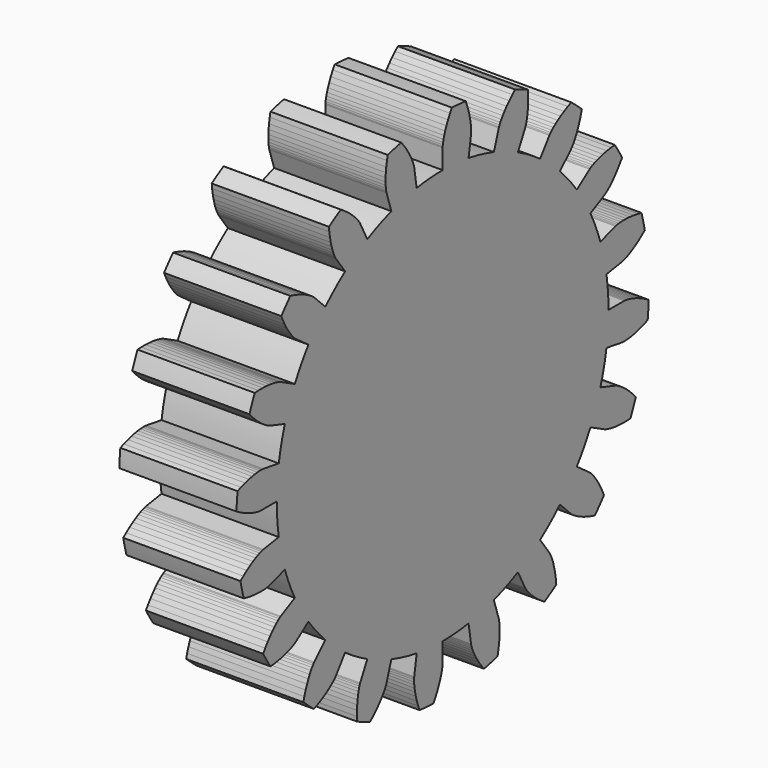
from build123d import *

# Parameters (mm, degrees)
F2_DEPTH = 12.7


# Not quite as in the source:
# - a variable given as a bare number and used for a length is read in inches; the dataset says mm whatever the document's units were


with BuildPart() as f2:
    # F1 (on Right) → F2 (new body)
    with BuildSketch(Plane.YZ):
        with BuildLine():
            ThreePointArc((22.1846851095, -3.5137089349), (22.3919795548, -1.7622870101), (22.46122, 0))
            ThreePointArc((22.46122, 0), (22.3919795548, 1.7622870101), (22.1846851095, 3.5137089349))
            ThreePointArc((22.1846851095, 3.5137089349), (21.8406147034, 5.2434676755), (21.3618896449, 6.9408986944))
            ThreePointArc((21.3618896449, 6.9408986944), (20.7514614332, 8.5955367647), (20.0130935612, 10.1971804926))
            ThreePointArc((20.0130935612, 10.1971804926), (19.1513383124, 11.7359552118), (18.1715086944, 13.2023738645))
            ThreePointArc((18.1715086944, 13.2023738645), (17.0796456827, 14.5873954921), (15.8824809757, 15.8824809757))
            ThreePointArc((15.8824809757, 15.8824809757), (14.5873954921, 17.0796456827), (13.2023738645, 18.1715086944))
            ThreePointArc((13.2023738645, 18.1715086944), (11.7359552118, 19.1513383124), (10.1971804926, 20.0130935612))
            ThreePointArc((10.1971804926, 20.0130935612), (8.5955367647, 20.7514614332), (6.9408986944, 21.3618896449))
            ThreePointArc((6.9408986944, 21.3618896449), (5.2434676755, 21.8406147034), (3.5137089349, 22.1846851095))
            ThreePointArc((3.5137089349, 22.1846851095), (1.7622870101, 22.3919795548), (0, 22.46122))
            ThreePointArc((0, 22.46122), (-1.7622870101, 22.3919795548), (-3.5137089349, 22.1846851095))
            ThreePointArc((-3.5137089349, 22.1846851095), (-5.2434676755, 21.8406147034), (-6.9408986944, 21.3618896449))
            ThreePointArc((-6.9408986944, 21.3618896449), (-8.5955367647, 20.7514614332), (-10.1971804926, 20.0130935612))
            ThreePointArc((-10.1971804926, 20.0130935612), (-11.7359552118, 19.1513383124), (-13.2023738645, 18.1715086944))
            ThreePointArc((-13.2023738645, 18.1715086944), (-14.5873954921, 17.0796456827), (-15.8824809757, 15.8824809757))
            ThreePointArc((-15.8824809757, 15.8824809757), (-17.0796456827, 14.5873954921), (-18.1715086944, 13.2023738645))
            ThreePointArc((-18.1715086944, 13.2023738645), (-19.1513383124, 11.7359552118), (-20.0130935612, 10.1971804926))
            ThreePointArc((-20.0130935612, 10.1971804926), (-20.7514614332, 8.5955367647), (-21.3618896449, 6.9408986944))
            ThreePointArc((-21.3618896449, 6.9408986944), (-21.8406147034, 5.2434676755), (-22.1846851095, 3.5137089349))
            ThreePointArc((-22.1846851095, 3.5137089349), (-22.3919795548, 1.7622870101), (-22.46122, 0))
            ThreePointArc((-22.46122, 0), (-22.3919795548, -1.7622870101), (-22.1846851095, -3.5137089349))
            ThreePointArc((-22.1846851095, -3.5137089349), (-21.8406147034, -5.2434676755), (-21.3618896449, -6.9408986944))
            ThreePointArc((-21.3618896449, -6.9408986944), (-20.7514614332, -8.5955367647), (-20.0130935612, -10.1971804926))
            ThreePointArc((-20.0130935612, -10.1971804926), (-19.1513383124, -11.7359552118), (-18.1715086944, -13.2023738645))
            ThreePointArc((-18.1715086944, -13.2023738645), (-17.0796456827, -14.5873954921), (-15.8824809757, -15.8824809757))
            ThreePointArc((-15.8824809757, -15.8824809757), (-14.5873954921, -17.0796456827), (-13.2023738645, -18.1715086944))
            ThreePointArc((-13.2023738645, -18.1715086944), (-11.7359552118, -19.1513383124), (-10.1971804926, -20.0130935612))
            ThreePointArc((-10.1971804926, -20.0130935612), (-8.5955367647, -20.7514614332), (-6.9408986944, -21.3618896449))
            ThreePointArc((-6.9408986944, -21.3618896449), (-5.2434676755, -21.8406147034), (-3.5137089349, -22.1846851095))
            ThreePointArc((-3.5137089349, -22.1846851095), (-1.7622870101, -22.3919795548), (0, -22.46122))
            ThreePointArc((0, -22.46122), (1.7622870101, -22.3919795548), (3.5137089349, -22.1846851095))
            ThreePointArc((3.5137089349, -22.1846851095), (5.2434676755, -21.8406147034), (6.9408986944, -21.3618896449))
            ThreePointArc((6.9408986944, -21.3618896449), (8.5955367647, -20.7514614332), (10.1971804926, -20.0130935612))
            ThreePointArc((10.1971804926, -20.0130935612), (11.7359552118, -19.1513383124), (13.2023738645, -18.1715086944))
            ThreePointArc((13.2023738645, -18.1715086944), (14.5873954921, -17.0796456827), (15.8824809757, -15.8824809757))
            ThreePointArc((15.8824809757, -15.8824809757), (17.0796456827, -14.5873954921), (18.1715086944, -13.2023738645))
            ThreePointArc((18.1715086944, -13.2023738645), (19.1513383124, -11.7359552118), (20.0130935612, -10.1971804926))
            ThreePointArc((20.0130935612, -10.1971804926), (20.7514614332, -8.5955367647), (21.3618896449, -6.9408986944))
            ThreePointArc((21.3618896449, -6.9408986944), (21.8406147034, -5.2434676755), (22.1846851095, -3.5137089349))
        make_face()
        with BuildLine():
            Line((-23.3873833018, -7.5990214781), (-21.3618896449, -6.9408986944))
            ThreePointArc((-21.3618896449, -6.9408986944), (-21.8406147034, -5.2434676755), (-22.1846851095, -3.5137089349))
            Line((-22.1846851095, -3.5137089349), (-24.288194664, -3.8468721183))
            Line((-24.288194664, -3.8468721183), (-24.3183756913, -3.8526894407))
            Line((-24.3183756913, -3.8526894407), (-24.4080512003, -3.8741463554))
            Line((-24.4080512003, -3.8741463554), (-24.5555837939, -3.9171690334))
            Line((-24.5555837939, -3.9171690334), (-24.7588943631, -3.987551636))
            Line((-24.7588943631, -3.987551636), (-25.0154715589, -4.0909270813))
            Line((-25.0154715589, -4.0909270813), (-25.3223830759, -4.2327384457))
            Line((-25.3223830759, -4.2327384457), (-25.6762887078, -4.4182111085))
            Line((-25.6762887078, -4.4182111085), (-26.0734551281, -4.6523257442))
            Line((-26.0734551281, -4.6523257442), (-26.5097723413, -4.939792266))
            Line((-26.5097723413, -4.939792266), (-26.9807717473, -5.2850248183))
            Line((-26.9807717473, -5.2850248183), (-27.3723694253, -5.6033018877))
            ThreePointArc((-27.3723694253, -5.6033018877), (-27.1680155759, -6.5224634661), (-26.9328055646, -7.4342171355))
            Line((-26.9328055646, -7.4342171355), (-26.4393947129, -7.5400224553))
            Line((-26.4393947129, -7.5400224553), (-25.8629988703, -7.633797656))
            Line((-25.8629988703, -7.633797656), (-25.3437303169, -7.6918483328))
            Line((-25.3437303169, -7.6918483328), (-24.8835666247, -7.720136219))
            Line((-24.8835666247, -7.720136219), (-24.4840315708, -7.7247237769))
            Line((-24.4840315708, -7.7247237769), (-24.1461903947, -7.7117437148))
            Line((-24.1461903947, -7.7117437148), (-23.8706469692, -7.6873683017))
            Line((-23.8706469692, -7.6873683017), (-23.6575428926, -7.6577785929))
            Line((-23.6575428926, -7.6577785929), (-23.5065585022, -7.6291336838))
            Line((-23.5065585022, -7.6291336838), (-23.4169158032, -7.6075401056))
            Line((-23.4169158032, -7.6075401056), (-23.3873833018, -7.5990214781))
        make_face()
        with BuildLine():
            Line((-19.8944965109, -14.4541977884), (-18.1715086944, -13.2023738645))
            ThreePointArc((-18.1715086944, -13.2023738645), (-19.1513383124, -11.7359552118), (-20.0130935612, -10.1971804926))
            Line((-20.0130935612, -10.1971804926), (-21.9106969444, -11.1640577094))
            Line((-21.9106969444, -11.1640577094), (-21.9376031557, -11.1789167621))
            Line((-21.9376031557, -11.1789167621), (-22.0162590816, -11.2270347569))
            Line((-22.0162590816, -11.2270347569), (-22.1432761774, -11.3135418337))
            Line((-22.1432761774, -11.3135418337), (-22.3148865988, -11.4433060876))
            Line((-22.3148865988, -11.4433060876), (-22.5269612434, -11.6209086924))
            Line((-22.5269612434, -11.6209086924), (-22.7750293199, -11.8506201891))
            Line((-22.7750293199, -11.8506201891), (-23.0542993726, -12.1363780283))
            Line((-23.0542993726, -12.1363780283), (-23.3596816836, -12.4817654516))
            Line((-23.3596816836, -12.4817654516), (-23.6858119718, -12.8899917942))
            Line((-23.6858119718, -12.8899917942), (-24.0270763004, -13.3638742835))
            Line((-24.0270763004, -13.3638742835), (-24.3011548004, -13.7875841018))
            ThreePointArc((-24.3011548004, -13.7875841018), (-23.8227661921, -14.5986098982), (-23.3173207996, -15.3930552759))
            Line((-23.3173207996, -15.3930552759), (-22.8153635519, -15.3412097764))
            Line((-22.8153635519, -15.3412097764), (-22.2382003992, -15.2522791813))
            Line((-22.2382003992, -15.2522791813), (-21.7264080121, -15.147025848))
            Line((-21.7264080121, -15.147025848), (-21.2800248965, -15.0317308255))
            Line((-21.2800248965, -15.0317308255), (-20.8986268467, -14.9126307308))
            Line((-20.8986268467, -14.9126307308), (-20.5813318544, -14.7958872934))
            Line((-20.5813318544, -14.7958872934), (-20.326806901, -14.6875572967))
            Line((-20.326806901, -14.6875572967), (-20.1332766032, -14.5935630301))
            Line((-20.1332766032, -14.5935630301), (-19.9985336785, -14.5196633601))
            Line((-19.9985336785, -14.5196633601), (-19.9199511881, -14.4714255295))
            Line((-19.9199511881, -14.4714255295), (-19.8944965109, -14.4541977884))
        make_face()
        with BuildLine():
            Line((-14.4541977884, -19.8944965109), (-13.2023738645, -18.1715086944))
            ThreePointArc((-13.2023738645, -18.1715086944), (-14.5873954921, -17.0796456827), (-15.8824809757, -15.8824809757))
            Line((-15.8824809757, -15.8824809757), (-17.3884275472, -17.3884275472))
            Line((-17.3884275472, -17.3884275472), (-17.409425175, -17.4108738227))
            Line((-17.409425175, -17.4108738227), (-17.4693621277, -17.480942773))
            Line((-17.4693621277, -17.480942773), (-17.5634304075, -17.6024663333))
            Line((-17.5634304075, -17.6024663333), (-17.6865422573, -17.7789100092))
            Line((-17.6865422573, -17.7789100092), (-17.8333550069, -18.013354793))
            Line((-17.8333550069, -18.013354793), (-17.9982970112, -18.3084806602))
            Line((-17.9982970112, -18.3084806602), (-18.175594586, -18.6665517076))
            Line((-18.175594586, -18.6665517076), (-18.3592998394, -19.0894029911))
            Line((-18.3592998394, -19.0894029911), (-18.5433192977, -19.5784291157))
            Line((-18.5433192977, -19.5784291157), (-18.7214432188, -20.1345746222))
            Line((-18.7214432188, -20.1345746222), (-18.8511738276, -20.6222415203))
            ThreePointArc((-18.8511738276, -20.6222415203), (-18.1455784703, -21.2457426789), (-17.4193742134, -21.8451139162))
            Line((-17.4193742134, -21.8451139162), (-16.9580056425, -21.6406925961))
            Line((-16.9580056425, -21.6406925961), (-16.4365719304, -21.3777613514))
            Line((-16.4365719304, -21.3777613514), (-15.9823535143, -21.1195069377))
            Line((-15.9823535143, -21.1195069377), (-15.5934460648, -20.8719148865))
            Line((-15.5934460648, -20.8719148865), (-15.2675189175, -20.6407854863))
            Line((-15.2675189175, -20.6407854863), (-15.0018291537, -20.4317063346))
            Line((-15.0018291537, -20.4317063346), (-14.7932373481, -20.2500258493))
            Line((-14.7932373481, -20.2500258493), (-14.6382249231, -20.1008278386))
            Line((-14.6382249231, -20.1008278386), (-14.5329130404, -19.9889072223))
            Line((-14.5329130404, -19.9889072223), (-14.4730829603, -19.9187469941))
            Line((-14.4730829603, -19.9187469941), (-14.4541977884, -19.8944965109))
        make_face()
        with BuildLine():
            Line((-7.5990214781, -23.3873833018), (-6.9408986944, -21.3618896449))
            ThreePointArc((-6.9408986944, -21.3618896449), (-8.5955367647, -20.7514614332), (-10.1971804926, -20.0130935612))
            Line((-10.1971804926, -20.0130935612), (-11.1640577094, -21.9106969444))
            Line((-11.1640577094, -21.9106969444), (-11.1770913595, -21.9385332448))
            Line((-11.1770913595, -21.9385332448), (-11.2124422925, -22.0236943136))
            Line((-11.2124422925, -22.0236943136), (-11.2643536976, -22.1683387846))
            Line((-11.2643536976, -22.1683387846), (-11.3269159302, -22.3741903461))
            Line((-11.3269159302, -22.3741903461), (-11.3940957299, -22.6425282201))
            Line((-11.3940957299, -22.6425282201), (-11.4597659895, -22.9741794817))
            Line((-11.4597659895, -22.9741794817), (-11.5177359646, -23.3695132482))
            Line((-11.5177359646, -23.3695132482), (-11.5617818102, -23.8284367621))
            Line((-11.5617818102, -23.8284367621), (-11.5856773319, -24.3503933845))
            Line((-11.5856773319, -24.3503933845), (-11.5832248349, -24.9343625111))
            Line((-11.5832248349, -24.9343625111), (-11.5559086167, -25.4382502551))
            ThreePointArc((-11.5559086167, -25.4382502551), (-10.6921751003, -25.8131941384), (-9.8162979113, -26.1588206026))
            Line((-9.8162979113, -26.1588206026), (-9.4406799874, -25.8218336449))
            Line((-9.4406799874, -25.8218336449), (-9.0260172807, -25.4106392928))
            Line((-9.0260172807, -25.4106392928), (-8.6738348989, -25.0246635401))
            Line((-8.6738348989, -25.0246635401), (-8.3804720864, -24.6690104953))
            Line((-8.3804720864, -24.6690104953), (-8.1419198617, -24.3484763457))
            Line((-8.1419198617, -24.3484763457), (-7.9538428915, -24.0675276037))
            Line((-7.9538428915, -24.0675276037), (-7.8116026531, -23.8302807815))
            Line((-7.8116026531, -23.8302807815), (-7.710281797, -23.6404835675))
            Line((-7.710281797, -23.6404835675), (-7.6447096172, -23.5014975746))
            Line((-7.6447096172, -23.5014975746), (-7.6094885324, -23.4162827209))
            Line((-7.6094885324, -23.4162827209), (-7.5990214781, -23.3873833018))
        make_face()
        with BuildLine():
            Line((0, -24.5909500656), (0, -22.46122))
            ThreePointArc((0, -22.46122), (-1.7622870101, -22.3919795548), (-3.5137089349, -22.1846851095))
            Line((-3.5137089349, -22.1846851095), (-3.8468721183, -24.288194664))
            Line((-3.8468721183, -24.288194664), (-3.8506659664, -24.3186961782))
            Line((-3.8506659664, -24.3186961782), (-3.8579704841, -24.4106132066))
            Line((-3.8579704841, -24.4106132066), (-3.8626435645, -24.5642197798))
            Line((-3.8626435645, -24.5642197798), (-3.8585321527, -24.7793290418))
            Line((-3.8585321527, -24.7793290418), (-3.8395029756, -25.0552932252))
            Line((-3.8395029756, -25.0552932252), (-3.7994732279, -25.3910055449))
            Line((-3.7994732279, -25.3910055449), (-3.7324410981, -25.7849040071))
            Line((-3.7324410981, -25.7849040071), (-3.6325160217, -26.2349771203))
            Line((-3.6325160217, -26.2349771203), (-3.4939485467, -26.7387714896))
            Line((-3.4939485467, -26.7387714896), (-3.3111596991, -27.2934012695))
            Line((-3.3111596991, -27.2934012695), (-3.1294705556, -27.7641858163))
            ThreePointArc((-3.1294705556, -27.7641858163), (-2.1921471346, -27.8538703045), (-1.2523339754, -27.9119196691))
            Line((-1.2523339754, -27.9119196691), (-0.9992347981, -27.4753537053))
            Line((-0.9992347981, -27.4753537053), (-0.7319331716, -26.9561468139))
            Line((-0.7319331716, -26.9561468139), (-0.5162608895, -26.4802317181))
            Line((-0.5162608895, -26.4802317181), (-0.3471591099, -26.0513314777))
            Line((-0.3471591099, -26.0513314777), (-0.2193329616, -25.6727686945))
            Line((-0.2193329616, -25.6727686945), (-0.1272790694, -25.3474515827))
            Line((-0.1272790694, -25.3474515827), (-0.0653138637, -25.0778617955))
            Line((-0.0653138637, -25.0778617955), (-0.0276025679, -24.8660440519))
            Line((-0.0276025679, -24.8660440519), (-0.0081887528, -24.7135975998))
            Line((-0.0081887528, -24.7135975998), (-0.0010243486, -24.6216695442))
            Line((-0.0010243486, -24.6216695442), (0, -24.5909500656))
        make_face()
        with BuildLine():
            Line((7.5990214781, -23.3873833018), (6.9408986944, -21.3618896449))
            ThreePointArc((6.9408986944, -21.3618896449), (5.2434676755, -21.8406147034), (3.5137089349, -22.1846851095))
            Line((3.5137089349, -22.1846851095), (3.8468721183, -24.288194664))
            Line((3.8468721183, -24.288194664), (3.8526894407, -24.3183756913))
            Line((3.8526894407, -24.3183756913), (3.8741463554, -24.4080512003))
            Line((3.8741463554, -24.4080512003), (3.9171690334, -24.5555837939))
            Line((3.9171690334, -24.5555837939), (3.987551636, -24.7588943631))
            Line((3.987551636, -24.7588943631), (4.0909270813, -25.0154715589))
            Line((4.0909270813, -25.0154715589), (4.2327384457, -25.3223830759))
            Line((4.2327384457, -25.3223830759), (4.4182111085, -25.6762887078))
            Line((4.4182111085, -25.6762887078), (4.6523257442, -26.0734551281))
            Line((4.6523257442, -26.0734551281), (4.939792266, -26.5097723413))
            Line((4.939792266, -26.5097723413), (5.2850248183, -26.9807717473))
            Line((5.2850248183, -26.9807717473), (5.6033018877, -27.3723694253))
            ThreePointArc((5.6033018877, -27.3723694253), (6.5224634661, -27.1680155759), (7.4342171355, -26.9328055646))
            Line((7.4342171355, -26.9328055646), (7.5400224553, -26.4393947129))
            Line((7.5400224553, -26.4393947129), (7.633797656, -25.8629988703))
            Line((7.633797656, -25.8629988703), (7.6918483328, -25.3437303169))
            Line((7.6918483328, -25.3437303169), (7.720136219, -24.8835666247))
            Line((7.720136219, -24.8835666247), (7.7247237769, -24.4840315708))
            Line((7.7247237769, -24.4840315708), (7.7117437148, -24.1461903947))
            Line((7.7117437148, -24.1461903947), (7.6873683017, -23.8706469692))
            Line((7.6873683017, -23.8706469692), (7.6577785929, -23.6575428926))
            Line((7.6577785929, -23.6575428926), (7.6291336838, -23.5065585022))
            Line((7.6291336838, -23.5065585022), (7.6075401056, -23.4169158032))
            Line((7.6075401056, -23.4169158032), (7.5990214781, -23.3873833018))
        make_face()
        with BuildLine():
            Line((14.4541977884, -19.8944965109), (13.2023738645, -18.1715086944))
            ThreePointArc((13.2023738645, -18.1715086944), (11.7359552118, -19.1513383124), (10.1971804926, -20.0130935612))
            Line((10.1971804926, -20.0130935612), (11.1640577094, -21.9106969444))
            Line((11.1640577094, -21.9106969444), (11.1789167621, -21.9376031557))
            Line((11.1789167621, -21.9376031557), (11.2270347569, -22.0162590816))
            Line((11.2270347569, -22.0162590816), (11.3135418337, -22.1432761774))
            Line((11.3135418337, -22.1432761774), (11.4433060876, -22.3148865988))
            Line((11.4433060876, -22.3148865988), (11.6209086924, -22.5269612434))
            Line((11.6209086924, -22.5269612434), (11.8506201891, -22.7750293199))
            Line((11.8506201891, -22.7750293199), (12.1363780283, -23.0542993726))
            Line((12.1363780283, -23.0542993726), (12.4817654516, -23.3596816836))
            Line((12.4817654516, -23.3596816836), (12.8899917942, -23.6858119718))
            Line((12.8899917942, -23.6858119718), (13.3638742835, -24.0270763004))
            Line((13.3638742835, -24.0270763004), (13.7875841018, -24.3011548004))
            ThreePointArc((13.7875841018, -24.3011548004), (14.5986098982, -23.8227661921), (15.3930552759, -23.3173207996))
            Line((15.3930552759, -23.3173207996), (15.3412097764, -22.8153635519))
            Line((15.3412097764, -22.8153635519), (15.2522791813, -22.2382003992))
            Line((15.2522791813, -22.2382003992), (15.147025848, -21.7264080121))
            Line((15.147025848, -21.7264080121), (15.0317308255, -21.2800248965))
            Line((15.0317308255, -21.2800248965), (14.9126307308, -20.8986268467))
            Line((14.9126307308, -20.8986268467), (14.7958872934, -20.5813318544))
            Line((14.7958872934, -20.5813318544), (14.6875572967, -20.326806901))
            Line((14.6875572967, -20.326806901), (14.5935630301, -20.1332766032))
            Line((14.5935630301, -20.1332766032), (14.5196633601, -19.9985336785))
            Line((14.5196633601, -19.9985336785), (14.4714255295, -19.9199511881))
            Line((14.4714255295, -19.9199511881), (14.4541977884, -19.8944965109))
        make_face()
        with BuildLine():
            Line((19.8944965109, -14.4541977884), (18.1715086944, -13.2023738645))
            ThreePointArc((18.1715086944, -13.2023738645), (17.0796456827, -14.5873954921), (15.8824809757, -15.8824809757))
            Line((15.8824809757, -15.8824809757), (17.3884275472, -17.3884275472))
            Line((17.3884275472, -17.3884275472), (17.4108738227, -17.409425175))
            Line((17.4108738227, -17.409425175), (17.480942773, -17.4693621277))
            Line((17.480942773, -17.4693621277), (17.6024663333, -17.5634304075))
            Line((17.6024663333, -17.5634304075), (17.7789100092, -17.6865422573))
            Line((17.7789100092, -17.6865422573), (18.013354793, -17.8333550069))
            Line((18.013354793, -17.8333550069), (18.3084806602, -17.9982970112))
            Line((18.3084806602, -17.9982970112), (18.6665517076, -18.175594586))
            Line((18.6665517076, -18.175594586), (19.0894029911, -18.3592998394))
            Line((19.0894029911, -18.3592998394), (19.5784291157, -18.5433192977))
            Line((19.5784291157, -18.5433192977), (20.1345746222, -18.7214432188))
            Line((20.1345746222, -18.7214432188), (20.6222415203, -18.8511738276))
            ThreePointArc((20.6222415203, -18.8511738276), (21.2457426789, -18.1455784703), (21.8451139162, -17.4193742134))
            Line((21.8451139162, -17.4193742134), (21.6406925961, -16.9580056425))
            Line((21.6406925961, -16.9580056425), (21.3777613514, -16.4365719304))
            Line((21.3777613514, -16.4365719304), (21.1195069377, -15.9823535143))
            Line((21.1195069377, -15.9823535143), (20.8719148865, -15.5934460648))
            Line((20.8719148865, -15.5934460648), (20.6407854863, -15.2675189175))
            Line((20.6407854863, -15.2675189175), (20.4317063346, -15.0018291537))
            Line((20.4317063346, -15.0018291537), (20.2500258493, -14.7932373481))
            Line((20.2500258493, -14.7932373481), (20.1008278386, -14.6382249231))
            Line((20.1008278386, -14.6382249231), (19.9889072223, -14.5329130404))
            Line((19.9889072223, -14.5329130404), (19.9187469941, -14.4730829603))
            Line((19.9187469941, -14.4730829603), (19.8944965109, -14.4541977884))
        make_face()
        with BuildLine():
            Line((23.3873833018, -7.5990214781), (21.3618896449, -6.9408986944))
            ThreePointArc((21.3618896449, -6.9408986944), (20.7514614332, -8.5955367647), (20.0130935612, -10.1971804926))
            Line((20.0130935612, -10.1971804926), (21.9106969444, -11.1640577094))
            Line((21.9106969444, -11.1640577094), (21.9385332448, -11.1770913595))
            Line((21.9385332448, -11.1770913595), (22.0236943136, -11.2124422925))
            Line((22.0236943136, -11.2124422925), (22.1683387846, -11.2643536976))
            Line((22.1683387846, -11.2643536976), (22.3741903461, -11.3269159302))
            Line((22.3741903461, -11.3269159302), (22.6425282201, -11.3940957299))
            Line((22.6425282201, -11.3940957299), (22.9741794817, -11.4597659895))
            Line((22.9741794817, -11.4597659895), (23.3695132482, -11.5177359646))
            Line((23.3695132482, -11.5177359646), (23.8284367621, -11.5617818102))
            Line((23.8284367621, -11.5617818102), (24.3503933845, -11.5856773319))
            Line((24.3503933845, -11.5856773319), (24.9343625111, -11.5832248349))
            Line((24.9343625111, -11.5832248349), (25.4382502551, -11.5559086167))
            ThreePointArc((25.4382502551, -11.5559086167), (25.8131941384, -10.6921751003), (26.1588206026, -9.8162979113))
            Line((26.1588206026, -9.8162979113), (25.8218336449, -9.4406799874))
            Line((25.8218336449, -9.4406799874), (25.4106392928, -9.0260172807))
            Line((25.4106392928, -9.0260172807), (25.0246635401, -8.6738348989))
            Line((25.0246635401, -8.6738348989), (24.6690104953, -8.3804720864))
            Line((24.6690104953, -8.3804720864), (24.3484763457, -8.1419198617))
            Line((24.3484763457, -8.1419198617), (24.0675276037, -7.9538428915))
            Line((24.0675276037, -7.9538428915), (23.8302807815, -7.8116026531))
            Line((23.8302807815, -7.8116026531), (23.6404835675, -7.710281797))
            Line((23.6404835675, -7.710281797), (23.5014975746, -7.6447096172))
            Line((23.5014975746, -7.6447096172), (23.4162827209, -7.6094885324))
            Line((23.4162827209, -7.6094885324), (23.3873833018, -7.5990214781))
        make_face()
        with BuildLine():
            Line((24.5909500656, 0), (22.46122, 0))
            ThreePointArc((22.46122, 0), (22.3919795548, -1.7622870101), (22.1846851095, -3.5137089349))
            Line((22.1846851095, -3.5137089349), (24.288194664, -3.8468721183))
            Line((24.288194664, -3.8468721183), (24.3186961782, -3.8506659664))
            Line((24.3186961782, -3.8506659664), (24.4106132066, -3.8579704841))
            Line((24.4106132066, -3.8579704841), (24.5642197798, -3.8626435645))
            Line((24.5642197798, -3.8626435645), (24.7793290418, -3.8585321527))
            Line((24.7793290418, -3.8585321527), (25.0552932252, -3.8395029756))
            Line((25.0552932252, -3.8395029756), (25.3910055449, -3.7994732279))
            Line((25.3910055449, -3.7994732279), (25.7849040071, -3.7324410981))
            Line((25.7849040071, -3.7324410981), (26.2349771203, -3.6325160217))
            Line((26.2349771203, -3.6325160217), (26.7387714896, -3.4939485467))
            Line((26.7387714896, -3.4939485467), (27.2934012695, -3.3111596991))
            Line((27.2934012695, -3.3111596991), (27.7641858163, -3.1294705556))
            ThreePointArc((27.7641858163, -3.1294705556), (27.8538703045, -2.1921471346), (27.9119196691, -1.2523339754))
            Line((27.9119196691, -1.2523339754), (27.4753537053, -0.9992347981))
            Line((27.4753537053, -0.9992347981), (26.9561468139, -0.7319331716))
            Line((26.9561468139, -0.7319331716), (26.4802317181, -0.5162608895))
            Line((26.4802317181, -0.5162608895), (26.0513314777, -0.3471591099))
            Line((26.0513314777, -0.3471591099), (25.6727686945, -0.2193329616))
            Line((25.6727686945, -0.2193329616), (25.3474515827, -0.1272790694))
            Line((25.3474515827, -0.1272790694), (25.0778617955, -0.0653138637))
            Line((25.0778617955, -0.0653138637), (24.8660440519, -0.0276025679))
            Line((24.8660440519, -0.0276025679), (24.7135975998, -0.0081887528))
            Line((24.7135975998, -0.0081887528), (24.6216695442, -0.0010243486))
            Line((24.6216695442, -0.0010243486), (24.5909500656, 0))
        make_face()
        with BuildLine():
            ThreePointArc((21.3618896449, 6.9408986944), (21.8406147034, 5.2434676755), (22.1846851095, 3.5137089349))
            Line((22.1846851095, 3.5137089349), (24.288194664, 3.8468721183))
            Line((24.288194664, 3.8468721183), (24.3183756913, 3.8526894407))
            Line((24.3183756913, 3.8526894407), (24.4080512003, 3.8741463554))
            Line((24.4080512003, 3.8741463554), (24.5555837939, 3.9171690334))
            Line((24.5555837939, 3.9171690334), (24.7588943631, 3.987551636))
            Line((24.7588943631, 3.987551636), (25.0154715589, 4.0909270813))
            Line((25.0154715589, 4.0909270813), (25.3223830759, 4.2327384457))
            Line((25.3223830759, 4.2327384457), (25.6762887078, 4.4182111085))
            Line((25.6762887078, 4.4182111085), (26.0734551281, 4.6523257442))
            Line((26.0734551281, 4.6523257442), (26.5097723413, 4.939792266))
            Line((26.5097723413, 4.939792266), (26.9807717473, 5.2850248183))
            Line((26.9807717473, 5.2850248183), (27.3723694253, 5.6033018877))
            ThreePointArc((27.3723694253, 5.6033018877), (27.1680155759, 6.5224634661), (26.9328055646, 7.4342171355))
            Line((26.9328055646, 7.4342171355), (26.4393947129, 7.5400224553))
            Line((26.4393947129, 7.5400224553), (25.8629988703, 7.633797656))
            Line((25.8629988703, 7.633797656), (25.3437303169, 7.6918483328))
            Line((25.3437303169, 7.6918483328), (24.8835666247, 7.720136219))
            Line((24.8835666247, 7.720136219), (24.4840315708, 7.7247237769))
            Line((24.4840315708, 7.7247237769), (24.1461903947, 7.7117437148))
            Line((24.1461903947, 7.7117437148), (23.8706469692, 7.6873683017))
            Line((23.8706469692, 7.6873683017), (23.6575428926, 7.6577785929))
            Line((23.6575428926, 7.6577785929), (23.5065585022, 7.6291336838))
            Line((23.5065585022, 7.6291336838), (23.4169158032, 7.6075401056))
            Line((23.4169158032, 7.6075401056), (23.3873833018, 7.5990214781))
            Line((23.3873833018, 7.5990214781), (21.3618896449, 6.9408986944))
        make_face()
        with BuildLine():
            ThreePointArc((18.1715086944, 13.2023738645), (19.1513383124, 11.7359552118), (20.0130935612, 10.1971804926))
            Line((20.0130935612, 10.1971804926), (21.9106969444, 11.1640577094))
            Line((21.9106969444, 11.1640577094), (21.9376031557, 11.1789167621))
            Line((21.9376031557, 11.1789167621), (22.0162590816, 11.2270347569))
            Line((22.0162590816, 11.2270347569), (22.1432761774, 11.3135418337))
            Line((22.1432761774, 11.3135418337), (22.3148865988, 11.4433060876))
            Line((22.3148865988, 11.4433060876), (22.5269612434, 11.6209086924))
            Line((22.5269612434, 11.6209086924), (22.7750293199, 11.8506201891))
            Line((22.7750293199, 11.8506201891), (23.0542993726, 12.1363780283))
            Line((23.0542993726, 12.1363780283), (23.3596816836, 12.4817654516))
            Line((23.3596816836, 12.4817654516), (23.6858119718, 12.8899917942))
            Line((23.6858119718, 12.8899917942), (24.0270763004, 13.3638742835))
            Line((24.0270763004, 13.3638742835), (24.3011548004, 13.7875841018))
            ThreePointArc((24.3011548004, 13.7875841018), (23.8227661921, 14.5986098982), (23.3173207996, 15.3930552759))
            Line((23.3173207996, 15.3930552759), (22.8153635519, 15.3412097764))
            Line((22.8153635519, 15.3412097764), (22.2382003992, 15.2522791813))
            Line((22.2382003992, 15.2522791813), (21.7264080121, 15.147025848))
            Line((21.7264080121, 15.147025848), (21.2800248965, 15.0317308255))
            Line((21.2800248965, 15.0317308255), (20.8986268467, 14.9126307308))
            Line((20.8986268467, 14.9126307308), (20.5813318544, 14.7958872934))
            Line((20.5813318544, 14.7958872934), (20.326806901, 14.6875572967))
            Line((20.326806901, 14.6875572967), (20.1332766032, 14.5935630301))
            Line((20.1332766032, 14.5935630301), (19.9985336785, 14.5196633601))
            Line((19.9985336785, 14.5196633601), (19.9199511881, 14.4714255295))
            Line((19.9199511881, 14.4714255295), (19.8944965109, 14.4541977884))
            Line((19.8944965109, 14.4541977884), (18.1715086944, 13.2023738645))
        make_face()
        with BuildLine():
            ThreePointArc((13.2023738645, 18.1715086944), (14.5873954921, 17.0796456827), (15.8824809757, 15.8824809757))
            Line((15.8824809757, 15.8824809757), (17.3884275472, 17.3884275472))
            Line((17.3884275472, 17.3884275472), (17.409425175, 17.4108738227))
            Line((17.409425175, 17.4108738227), (17.4693621277, 17.480942773))
            Line((17.4693621277, 17.480942773), (17.5634304075, 17.6024663333))
            Line((17.5634304075, 17.6024663333), (17.6865422573, 17.7789100092))
            Line((17.6865422573, 17.7789100092), (17.8333550069, 18.013354793))
            Line((17.8333550069, 18.013354793), (17.9982970112, 18.3084806602))
            Line((17.9982970112, 18.3084806602), (18.175594586, 18.6665517076))
            Line((18.175594586, 18.6665517076), (18.3592998394, 19.0894029911))
            Line((18.3592998394, 19.0894029911), (18.5433192977, 19.5784291157))
            Line((18.5433192977, 19.5784291157), (18.7214432188, 20.1345746222))
            Line((18.7214432188, 20.1345746222), (18.8511738276, 20.6222415203))
            ThreePointArc((18.8511738276, 20.6222415203), (18.1455784703, 21.2457426789), (17.4193742134, 21.8451139162))
            Line((17.4193742134, 21.8451139162), (16.9580056425, 21.6406925961))
            Line((16.9580056425, 21.6406925961), (16.4365719304, 21.3777613514))
            Line((16.4365719304, 21.3777613514), (15.9823535143, 21.1195069377))
            Line((15.9823535143, 21.1195069377), (15.5934460648, 20.8719148865))
            Line((15.5934460648, 20.8719148865), (15.2675189175, 20.6407854863))
            Line((15.2675189175, 20.6407854863), (15.0018291537, 20.4317063346))
            Line((15.0018291537, 20.4317063346), (14.7932373481, 20.2500258493))
            Line((14.7932373481, 20.2500258493), (14.6382249231, 20.1008278386))
            Line((14.6382249231, 20.1008278386), (14.5329130404, 19.9889072223))
            Line((14.5329130404, 19.9889072223), (14.4730829603, 19.9187469941))
            Line((14.4730829603, 19.9187469941), (14.4541977884, 19.8944965109))
            Line((14.4541977884, 19.8944965109), (13.2023738645, 18.1715086944))
        make_face()
        with BuildLine():
            ThreePointArc((6.9408986944, 21.3618896449), (8.5955367647, 20.7514614332), (10.1971804926, 20.0130935612))
            Line((10.1971804926, 20.0130935612), (11.1640577094, 21.9106969444))
            Line((11.1640577094, 21.9106969444), (11.1770913595, 21.9385332448))
            Line((11.1770913595, 21.9385332448), (11.2124422925, 22.0236943136))
            Line((11.2124422925, 22.0236943136), (11.2643536976, 22.1683387846))
            Line((11.2643536976, 22.1683387846), (11.3269159302, 22.3741903461))
            Line((11.3269159302, 22.3741903461), (11.3940957299, 22.6425282201))
            Line((11.3940957299, 22.6425282201), (11.4597659895, 22.9741794817))
            Line((11.4597659895, 22.9741794817), (11.5177359646, 23.3695132482))
            Line((11.5177359646, 23.3695132482), (11.5617818102, 23.8284367621))
            Line((11.5617818102, 23.8284367621), (11.5856773319, 24.3503933845))
            Line((11.5856773319, 24.3503933845), (11.5832248349, 24.9343625111))
            Line((11.5832248349, 24.9343625111), (11.5559086167, 25.4382502551))
            ThreePointArc((11.5559086167, 25.4382502551), (10.6921751003, 25.8131941384), (9.8162979113, 26.1588206026))
            Line((9.8162979113, 26.1588206026), (9.4406799874, 25.8218336449))
            Line((9.4406799874, 25.8218336449), (9.0260172807, 25.4106392928))
            Line((9.0260172807, 25.4106392928), (8.6738348989, 25.0246635401))
            Line((8.6738348989, 25.0246635401), (8.3804720864, 24.6690104953))
            Line((8.3804720864, 24.6690104953), (8.1419198617, 24.3484763457))
            Line((8.1419198617, 24.3484763457), (7.9538428915, 24.0675276037))
            Line((7.9538428915, 24.0675276037), (7.8116026531, 23.8302807815))
            Line((7.8116026531, 23.8302807815), (7.710281797, 23.6404835675))
            Line((7.710281797, 23.6404835675), (7.6447096172, 23.5014975746))
            Line((7.6447096172, 23.5014975746), (7.6094885324, 23.4162827209))
            Line((7.6094885324, 23.4162827209), (7.5990214781, 23.3873833018))
            Line((7.5990214781, 23.3873833018), (6.9408986944, 21.3618896449))
        make_face()
        with BuildLine():
            ThreePointArc((0, 22.46122), (1.7622870101, 22.3919795548), (3.5137089349, 22.1846851095))
            Line((3.5137089349, 22.1846851095), (3.8468721183, 24.288194664))
            Line((3.8468721183, 24.288194664), (3.8506659664, 24.3186961782))
            Line((3.8506659664, 24.3186961782), (3.8579704841, 24.4106132066))
            Line((3.8579704841, 24.4106132066), (3.8626435645, 24.5642197798))
            Line((3.8626435645, 24.5642197798), (3.8585321527, 24.7793290418))
            Line((3.8585321527, 24.7793290418), (3.8395029756, 25.0552932252))
            Line((3.8395029756, 25.0552932252), (3.7994732279, 25.3910055449))
            Line((3.7994732279, 25.3910055449), (3.7324410981, 25.7849040071))
            Line((3.7324410981, 25.7849040071), (3.6325160217, 26.2349771203))
            Line((3.6325160217, 26.2349771203), (3.4939485467, 26.7387714896))
            Line((3.4939485467, 26.7387714896), (3.3111596991, 27.2934012695))
            Line((3.3111596991, 27.2934012695), (3.1294705556, 27.7641858163))
            ThreePointArc((3.1294705556, 27.7641858163), (2.1921471346, 27.8538703045), (1.2523339754, 27.9119196691))
            Line((1.2523339754, 27.9119196691), (0.9992347981, 27.4753537053))
            Line((0.9992347981, 27.4753537053), (0.7319331716, 26.9561468139))
            Line((0.7319331716, 26.9561468139), (0.5162608895, 26.4802317181))
            Line((0.5162608895, 26.4802317181), (0.3471591099, 26.0513314777))
            Line((0.3471591099, 26.0513314777), (0.2193329616, 25.6727686945))
            Line((0.2193329616, 25.6727686945), (0.1272790694, 25.3474515827))
            Line((0.1272790694, 25.3474515827), (0.0653138637, 25.0778617955))
            Line((0.0653138637, 25.0778617955), (0.0276025679, 24.8660440519))
            Line((0.0276025679, 24.8660440519), (0.0081887528, 24.7135975998))
            Line((0.0081887528, 24.7135975998), (0.0010243486, 24.6216695442))
            Line((0.0010243486, 24.6216695442), (0, 24.5909500656))
            Line((0, 24.5909500656), (0, 22.46122))
        make_face()
        with BuildLine():
            ThreePointArc((-6.9408986944, 21.3618896449), (-5.2434676755, 21.8406147034), (-3.5137089349, 22.1846851095))
            Line((-3.5137089349, 22.1846851095), (-3.8468721183, 24.288194664))
            Line((-3.8468721183, 24.288194664), (-3.8526894407, 24.3183756913))
            Line((-3.8526894407, 24.3183756913), (-3.8741463554, 24.4080512003))
            Line((-3.8741463554, 24.4080512003), (-3.9171690334, 24.5555837939))
            Line((-3.9171690334, 24.5555837939), (-3.987551636, 24.7588943631))
            Line((-3.987551636, 24.7588943631), (-4.0909270813, 25.0154715589))
            Line((-4.0909270813, 25.0154715589), (-4.2327384457, 25.3223830759))
            Line((-4.2327384457, 25.3223830759), (-4.4182111085, 25.6762887078))
            Line((-4.4182111085, 25.6762887078), (-4.6523257442, 26.0734551281))
            Line((-4.6523257442, 26.0734551281), (-4.939792266, 26.5097723413))
            Line((-4.939792266, 26.5097723413), (-5.2850248183, 26.9807717473))
            Line((-5.2850248183, 26.9807717473), (-5.6033018877, 27.3723694253))
            ThreePointArc((-5.6033018877, 27.3723694253), (-6.5224634661, 27.1680155759), (-7.4342171355, 26.9328055646))
            Line((-7.4342171355, 26.9328055646), (-7.5400224553, 26.4393947129))
            Line((-7.5400224553, 26.4393947129), (-7.633797656, 25.8629988703))
            Line((-7.633797656, 25.8629988703), (-7.6918483328, 25.3437303169))
            Line((-7.6918483328, 25.3437303169), (-7.720136219, 24.8835666247))
            Line((-7.720136219, 24.8835666247), (-7.7247237769, 24.4840315708))
            Line((-7.7247237769, 24.4840315708), (-7.7117437148, 24.1461903947))
            Line((-7.7117437148, 24.1461903947), (-7.6873683017, 23.8706469692))
            Line((-7.6873683017, 23.8706469692), (-7.6577785929, 23.6575428926))
            Line((-7.6577785929, 23.6575428926), (-7.6291336838, 23.5065585022))
            Line((-7.6291336838, 23.5065585022), (-7.6075401056, 23.4169158032))
            Line((-7.6075401056, 23.4169158032), (-7.5990214781, 23.3873833018))
            Line((-7.5990214781, 23.3873833018), (-6.9408986944, 21.3618896449))
        make_face()
        with BuildLine():
            ThreePointArc((-13.2023738645, 18.1715086944), (-11.7359552118, 19.1513383124), (-10.1971804926, 20.0130935612))
            Line((-10.1971804926, 20.0130935612), (-11.1640577094, 21.9106969444))
            Line((-11.1640577094, 21.9106969444), (-11.1789167621, 21.9376031557))
            Line((-11.1789167621, 21.9376031557), (-11.2270347569, 22.0162590816))
            Line((-11.2270347569, 22.0162590816), (-11.3135418337, 22.1432761774))
            Line((-11.3135418337, 22.1432761774), (-11.4433060876, 22.3148865988))
            Line((-11.4433060876, 22.3148865988), (-11.6209086924, 22.5269612434))
            Line((-11.6209086924, 22.5269612434), (-11.8506201891, 22.7750293199))
            Line((-11.8506201891, 22.7750293199), (-12.1363780283, 23.0542993726))
            Line((-12.1363780283, 23.0542993726), (-12.4817654516, 23.3596816836))
            Line((-12.4817654516, 23.3596816836), (-12.8899917942, 23.6858119718))
            Line((-12.8899917942, 23.6858119718), (-13.3638742835, 24.0270763004))
            Line((-13.3638742835, 24.0270763004), (-13.7875841018, 24.3011548004))
            ThreePointArc((-13.7875841018, 24.3011548004), (-14.5986098982, 23.8227661921), (-15.3930552759, 23.3173207996))
            Line((-15.3930552759, 23.3173207996), (-15.3412097764, 22.8153635519))
            Line((-15.3412097764, 22.8153635519), (-15.2522791813, 22.2382003992))
            Line((-15.2522791813, 22.2382003992), (-15.147025848, 21.7264080121))
            Line((-15.147025848, 21.7264080121), (-15.0317308255, 21.2800248965))
            Line((-15.0317308255, 21.2800248965), (-14.9126307308, 20.8986268467))
            Line((-14.9126307308, 20.8986268467), (-14.7958872934, 20.5813318544))
            Line((-14.7958872934, 20.5813318544), (-14.6875572967, 20.326806901))
            Line((-14.6875572967, 20.326806901), (-14.5935630301, 20.1332766032))
            Line((-14.5935630301, 20.1332766032), (-14.5196633601, 19.9985336785))
            Line((-14.5196633601, 19.9985336785), (-14.4714255295, 19.9199511881))
            Line((-14.4714255295, 19.9199511881), (-14.4541977884, 19.8944965109))
            Line((-14.4541977884, 19.8944965109), (-13.2023738645, 18.1715086944))
        make_face()
        with BuildLine():
            ThreePointArc((-18.1715086944, 13.2023738645), (-17.0796456827, 14.5873954921), (-15.8824809757, 15.8824809757))
            Line((-15.8824809757, 15.8824809757), (-17.3884275472, 17.3884275472))
            Line((-17.3884275472, 17.3884275472), (-17.4108738227, 17.409425175))
            Line((-17.4108738227, 17.409425175), (-17.480942773, 17.4693621277))
            Line((-17.480942773, 17.4693621277), (-17.6024663333, 17.5634304075))
            Line((-17.6024663333, 17.5634304075), (-17.7789100092, 17.6865422573))
            Line((-17.7789100092, 17.6865422573), (-18.013354793, 17.8333550069))
            Line((-18.013354793, 17.8333550069), (-18.3084806602, 17.9982970112))
            Line((-18.3084806602, 17.9982970112), (-18.6665517076, 18.175594586))
            Line((-18.6665517076, 18.175594586), (-19.0894029911, 18.3592998394))
            Line((-19.0894029911, 18.3592998394), (-19.5784291157, 18.5433192977))
            Line((-19.5784291157, 18.5433192977), (-20.1345746222, 18.7214432188))
            Line((-20.1345746222, 18.7214432188), (-20.6222415203, 18.8511738276))
            ThreePointArc((-20.6222415203, 18.8511738276), (-21.2457426789, 18.1455784703), (-21.8451139162, 17.4193742134))
            Line((-21.8451139162, 17.4193742134), (-21.6406925961, 16.9580056425))
            Line((-21.6406925961, 16.9580056425), (-21.3777613514, 16.4365719304))
            Line((-21.3777613514, 16.4365719304), (-21.1195069377, 15.9823535143))
            Line((-21.1195069377, 15.9823535143), (-20.8719148865, 15.5934460648))
            Line((-20.8719148865, 15.5934460648), (-20.6407854863, 15.2675189175))
            Line((-20.6407854863, 15.2675189175), (-20.4317063346, 15.0018291537))
            Line((-20.4317063346, 15.0018291537), (-20.2500258493, 14.7932373481))
            Line((-20.2500258493, 14.7932373481), (-20.1008278386, 14.6382249231))
            Line((-20.1008278386, 14.6382249231), (-19.9889072223, 14.5329130404))
            Line((-19.9889072223, 14.5329130404), (-19.9187469941, 14.4730829603))
            Line((-19.9187469941, 14.4730829603), (-19.8944965109, 14.4541977884))
            Line((-19.8944965109, 14.4541977884), (-18.1715086944, 13.2023738645))
        make_face()
        with BuildLine():
            ThreePointArc((-21.3618896449, 6.9408986944), (-20.7514614332, 8.5955367647), (-20.0130935612, 10.1971804926))
            Line((-20.0130935612, 10.1971804926), (-21.9106969444, 11.1640577094))
            Line((-21.9106969444, 11.1640577094), (-21.9385332448, 11.1770913595))
            Line((-21.9385332448, 11.1770913595), (-22.0236943136, 11.2124422925))
            Line((-22.0236943136, 11.2124422925), (-22.1683387846, 11.2643536976))
            Line((-22.1683387846, 11.2643536976), (-22.3741903461, 11.3269159302))
            Line((-22.3741903461, 11.3269159302), (-22.6425282201, 11.3940957299))
            Line((-22.6425282201, 11.3940957299), (-22.9741794817, 11.4597659895))
            Line((-22.9741794817, 11.4597659895), (-23.3695132482, 11.5177359646))
            Line((-23.3695132482, 11.5177359646), (-23.8284367621, 11.5617818102))
            Line((-23.8284367621, 11.5617818102), (-24.3503933845, 11.5856773319))
            Line((-24.3503933845, 11.5856773319), (-24.9343625111, 11.5832248349))
            Line((-24.9343625111, 11.5832248349), (-25.4382502551, 11.5559086167))
            ThreePointArc((-25.4382502551, 11.5559086167), (-25.8131941384, 10.6921751003), (-26.1588206026, 9.8162979113))
            Line((-26.1588206026, 9.8162979113), (-25.8218336449, 9.4406799874))
            Line((-25.8218336449, 9.4406799874), (-25.4106392928, 9.0260172807))
            Line((-25.4106392928, 9.0260172807), (-25.0246635401, 8.6738348989))
            Line((-25.0246635401, 8.6738348989), (-24.6690104953, 8.3804720864))
            Line((-24.6690104953, 8.3804720864), (-24.3484763457, 8.1419198617))
            Line((-24.3484763457, 8.1419198617), (-24.0675276037, 7.9538428915))
            Line((-24.0675276037, 7.9538428915), (-23.8302807815, 7.8116026531))
            Line((-23.8302807815, 7.8116026531), (-23.6404835675, 7.710281797))
            Line((-23.6404835675, 7.710281797), (-23.5014975746, 7.6447096172))
            Line((-23.5014975746, 7.6447096172), (-23.4162827209, 7.6094885324))
            Line((-23.4162827209, 7.6094885324), (-23.3873833018, 7.5990214781))
            Line((-23.3873833018, 7.5990214781), (-21.3618896449, 6.9408986944))
        make_face()
        with BuildLine():
            ThreePointArc((-22.46122, 0), (-22.3919795548, 1.7622870101), (-22.1846851095, 3.5137089349))
            Line((-22.1846851095, 3.5137089349), (-24.288194664, 3.8468721183))
            Line((-24.288194664, 3.8468721183), (-24.3186961782, 3.8506659664))
            Line((-24.3186961782, 3.8506659664), (-24.4106132066, 3.8579704841))
            Line((-24.4106132066, 3.8579704841), (-24.5642197798, 3.8626435645))
            Line((-24.5642197798, 3.8626435645), (-24.7793290418, 3.8585321527))
            Line((-24.7793290418, 3.8585321527), (-25.0552932252, 3.8395029756))
            Line((-25.0552932252, 3.8395029756), (-25.3910055449, 3.7994732279))
            Line((-25.3910055449, 3.7994732279), (-25.7849040071, 3.7324410981))
            Line((-25.7849040071, 3.7324410981), (-26.2349771203, 3.6325160217))
            Line((-26.2349771203, 3.6325160217), (-26.7387714896, 3.4939485467))
            Line((-26.7387714896, 3.4939485467), (-27.2934012695, 3.3111596991))
            Line((-27.2934012695, 3.3111596991), (-27.7641858163, 3.1294705556))
            ThreePointArc((-27.7641858163, 3.1294705556), (-27.8538703045, 2.1921471346), (-27.9119196691, 1.2523339754))
            Line((-27.9119196691, 1.2523339754), (-27.4753537053, 0.9992347981))
            Line((-27.4753537053, 0.9992347981), (-26.9561468139, 0.7319331716))
            Line((-26.9561468139, 0.7319331716), (-26.4802317181, 0.5162608895))
            Line((-26.4802317181, 0.5162608895), (-26.0513314777, 0.3471591099))
            Line((-26.0513314777, 0.3471591099), (-25.6727686945, 0.2193329616))
            Line((-25.6727686945, 0.2193329616), (-25.3474515827, 0.1272790694))
            Line((-25.3474515827, 0.1272790694), (-25.0778617955, 0.0653138637))
            Line((-25.0778617955, 0.0653138637), (-24.8660440519, 0.0276025679))
            Line((-24.8660440519, 0.0276025679), (-24.7135975998, 0.0081887528))
            Line((-24.7135975998, 0.0081887528), (-24.6216695442, 0.0010243486))
            Line((-24.6216695442, 0.0010243486), (-24.5909500656, 0))
            Line((-24.5909500656, 0), (-22.46122, 0))
        make_face()
    extrude(amount=F2_DEPTH)


solid = f2.part
